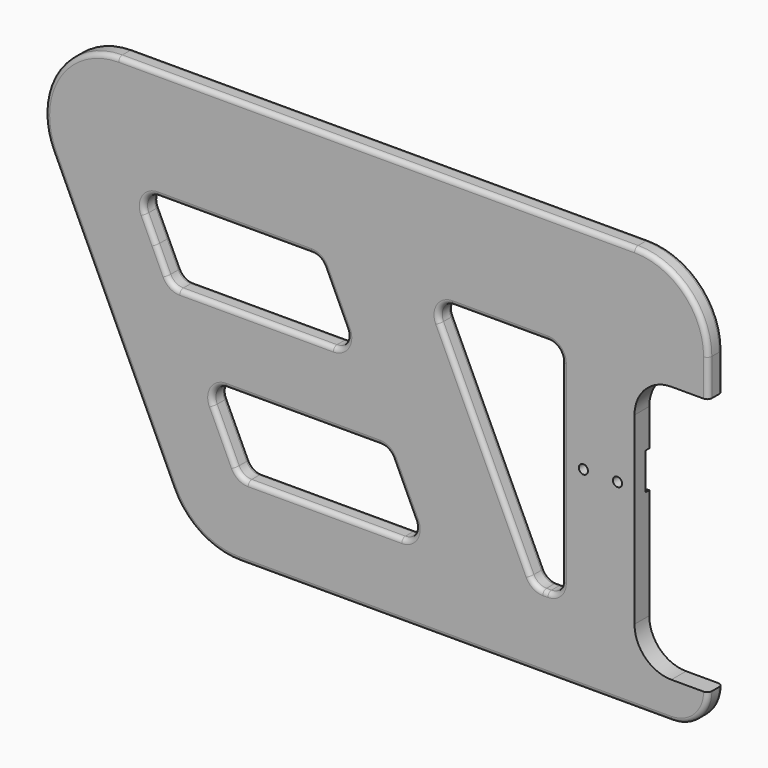
from build123d import *

# Parameters (mm, degrees)
F1_DEPTH = 6.35
F2_R     = 1.5875
F3_R     = 1.5875
F4_DEPTH = 25.4
F6_DEPTH = 1.5875


# Not quite as in the source:
# - a feature names something its author has since deleted; it is built from what else it names


with BuildPart() as f1:
    # F0 (on Front) → F1 (new body)
    with BuildSketch(Plane.XZ):
        with BuildLine():
            ThreePointArc((114.3, 44.45), (106.8605122421, 62.4105122421), (88.9, 69.85))
            Line((88.9, 69.85), (0, 69.85))
            Line((0, 69.85), (-88.9, 69.85))
            ThreePointArc((-88.9, 69.85), (-106.8605122421, 62.4105122421), (-114.3, 44.45))
            ThreePointArc((-114.3, 44.45), (-113.6951513287, 38.9399663714), (-111.9094117647, 33.6923529412))
            Line((-111.9094117647, 33.6923529412), (-70.3457754011, -55.2076470588))
            ThreePointArc((-70.3457754011, -55.2076470588), (-60.9730011381, -65.8790017884), (-47.3363636364, -69.85))
            Line((-47.3363636364, -69.85), (101.6, -69.85))
            ThreePointArc((101.6, -69.85), (110.5802561211, -66.1302561211), (114.3, -57.15))
            Line((114.3, -57.15), (101.6, -57.15))
            ThreePointArc((101.6, -57.15), (92.6197438789, -53.4302561211), (88.9, -44.45))
            Line((88.9, -44.45), (88.9, 19.05))
            ThreePointArc((88.9, 19.05), (92.6197438789, 28.0302561211), (101.6, 31.75))
            Line((101.6, 31.75), (114.3, 31.75))
            Line((114.3, 31.75), (114.3, 44.45))
        make_face()
        with BuildLine():
            Line((8.6597506493, -44.45), (-44.2976, -44.45))
            ThreePointArc((-44.2976, -44.45), (-46.8612878503, -43.7034523362), (-48.6233694118, -41.6972376471))
            Line((-48.6233694118, -41.6972376471), (-56.2029001681, -25.4854635294))
            ThreePointArc((-56.2029001681, -25.4854635294), (-55.9057830925, -20.899338032), (-51.8771307563, -18.6878258824))
            Line((-51.8771307563, -18.6878258824), (1.080219893, -18.6878258824))
            ThreePointArc((1.080219893, -18.6878258824), (3.6439077434, -19.4343735461), (5.4059893048, -21.4405882353))
            Line((5.4059893048, -21.4405882353), (12.9855200611, -37.6523623529))
            ThreePointArc((12.9855200611, -37.6523623529), (12.6884029856, -42.2384878503), (8.6597506493, -44.45))
        make_face(mode=Mode.SUBTRACT)
        with BuildLine():
            Line((52.9766305882, -41.6972376471), (21.8157786402, 24.9523623529))
            ThreePointArc((21.8157786402, 24.9523623529), (22.1128957157, 29.5384878503), (26.1415480519, 31.75))
            Line((26.1415480519, 31.75), (59.0388363636, 31.75))
            ThreePointArc((59.0388363636, 31.75), (62.4154126652, 30.3513763015), (63.8140363636, 26.9748))
            Line((63.8140363636, 26.9748), (63.8140363636, -39.6748))
            ThreePointArc((63.8140363636, -39.6748), (62.4154126652, -43.0513763015), (59.0388363636, -44.45))
            Line((59.0388363636, -44.45), (57.3024, -44.45))
            ThreePointArc((57.3024, -44.45), (54.7387121497, -43.7034523362), (52.9766305882, -41.6972376471))
        make_face(mode=Mode.SUBTRACT)
        with BuildLine():
            Line((-75.4584519481, 31.75), (-46.5189740062, 31.75))
            Line((-46.5189740062, 31.75), (-22.5011012987, 31.75))
            ThreePointArc((-22.5011012987, 31.75), (-19.9374134484, 31.0034523362), (-18.1753318869, 28.9972376471))
            Line((-18.1753318869, 28.9972376471), (-10.595799035, 12.7854590471))
            ThreePointArc((-10.595799035, 12.7854590471), (-10.8929161105, 8.1993335497), (-14.9215684468, 5.9878214))
            Line((-14.9215684468, 5.9878214), (-67.8789190961, 5.9878214))
            ThreePointArc((-67.8789190961, 5.9878214), (-70.4426069464, 6.7343690638), (-72.2046885079, 8.7405837529))
            Line((-72.2046885079, 8.7405837529), (-76.0224587934, 16.906370197))
            Line((-76.0224587934, 16.906370197), (-79.7842213598, 24.9523623529))
            ThreePointArc((-79.7842213598, 24.9523623529), (-79.4871042843, 29.5384878503), (-75.4584519481, 31.75))
        make_face(mode=Mode.SUBTRACT)
    extrude(amount=F1_DEPTH)

    # F2
    f2_edges = [f1.edges().sort_by_distance(p)[0] for p in [
        (-91.127594, -6.35, -10.757647),
        (27.131818, 0, -69.85),
        (-25.398455, -6.35, -18.687826),
        (42.590192, 0, 31.75),
        (-25.398455, 0, -18.687826),
        (-48.979777, -6.35, 31.75),
        (42.590192, -6.35, 31.75),
        (-48.979777, 0, 31.75),
    ]]
    fillet(f2_edges, radius=F2_R)

    # F3 (on face) → F4 (cut)
    with BuildSketch(Plane(origin=(0, 0, 0), x_dir=(-1, 0, 0), z_dir=(0, 1, 0))):
        with Locations((-83.0253840909, -3.175)):
            Circle(F3_R)
        with Locations((-71.2761522727, -3.175)):
            Circle(F3_R)
    extrude(amount=-F4_DEPTH, mode=Mode.SUBTRACT)

    # F5 (on face) → F6 (cut)
    with BuildSketch(Plane(origin=(0, 0, 0), x_dir=(-1, 0, 0), z_dir=(0, 1, 0))):
        Polygon((-65.4015363636, 6.35), (-88.9, 6.35), (-88.9, -6.35), (-65.4015363636, -6.35), (-61.6288669407, -6.35), (-61.6288669407, 6.35), align=None)
    extrude(amount=-F6_DEPTH, mode=Mode.SUBTRACT)


solid = f1.part
